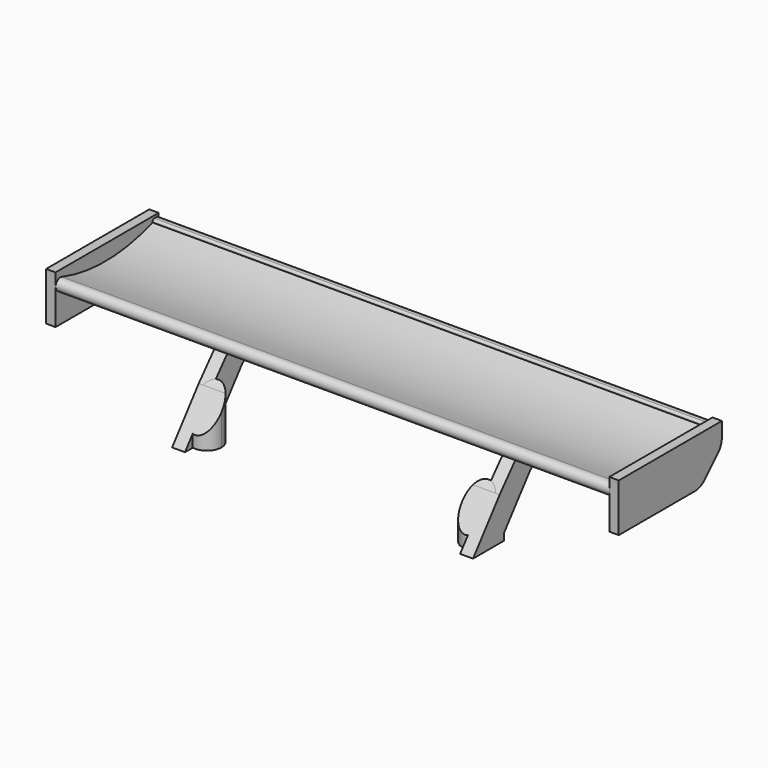
from build123d import *

# Parameters (mm, degrees)
F4_W      = 15
F4_H      = 5.6
F5_DEPTH  = 1.1
F6_SIZE   = 3.1
F7_W      = 15
F7_H      = 5.6
F8_DEPTH  = 1.1
F9_SIZE   = 3.1
F11_DEPTH = 32.2
F12_R     = 0.25
F13_R     = 2
F15_DEPTH = 1.5
F17_DEPTH = 1.5
F18_R     = 1.7
F19_DEPTH = 6.8
F22_W     = 36
F22_H     = 4
F24_R     = 0.75
F25_DEPTH = 2.5


with BuildPart() as f5:
    # F4 (on offset) → F5 (new body)
    with BuildSketch(Plane.YZ.offset(33.3)):
        with Locations((7.5, 2.8)):
            Rectangle(F4_W, F4_H)
    extrude(amount=-F5_DEPTH)

    # F6
    f6_edges = [f5.edges().sort_by_distance(p)[0] for p in [
        (32.75, 15, 0),
    ]]
    chamfer(f6_edges, length=F6_SIZE)



with BuildPart() as f8:
    # F7 (on offset) → F8 (new body)
    with BuildSketch(Plane.YZ.offset(-33.3)):
        with Locations((7.5, 2.8)):
            Rectangle(F7_W, F7_H)
    extrude(amount=F8_DEPTH)

    # F9
    f9_edges = [f8.edges().sort_by_distance(p)[0] for p in [
        (-32.75, 15, 0),
    ]]
    chamfer(f9_edges, length=F9_SIZE)


with BuildPart() as f5_1:
    add(f5.part)

    add(f8.part)  # F11 merges F8
    # F10 (on Right) → F11 (join, symmetric)
    with BuildSketch(Plane.YZ):
        with BuildLine():
            ThreePointArc((14.1, 4.9799904701), (7.5241974898, 3.7896224533), (0.9153141097, 4.7799835677))
            ThreePointArc((0.9153141097, 4.7799835677), (0.075756099, 4.4131641565), (0.3380033304, 3.5353028215))
            ThreePointArc((0.3380033304, 3.5353028215), (0.8766544844, 3.272139492), (1.4572901418, 3.1229341403))
            ThreePointArc((1.4572901418, 3.1229341403), (7.8107981998, 2.7603942388), (14.0573066811, 3.9767953297))
            ThreePointArc((14.0573066811, 3.9767953297), (14.7402257131, 4.4876667413), (15, 5.3))
            Line((15, 5.3), (14.1, 5.3))
            Line((14.1, 5.3), (14.1, 4.9799904701))
        make_face()
    extrude(amount=F11_DEPTH, both=True)

    # F12
    f12_edges = [f5_1.edges().sort_by_distance(p)[0] for p in [
        (0, 14.1, 5.3),
        (0, 15, 5.3),
    ]]
    fillet(f12_edges, radius=F12_R)

    # F13
    f13_edges = [f5_1.edges().sort_by_distance(p)[0] for p in [
        (32.75, 11.9, 0),
        (32.75, 15, 3.1),
        (-32.75, 15, 3.1),
        (-32.75, 11.9, 0),
    ]]
    fillet(f13_edges, radius=F13_R)

    # F14 (on offset) → F15 (join)
    with BuildSketch(Plane.YZ.offset(-16)):
        with BuildLine():
            ThreePointArc((10, 3.0037642772), (7.4076873546, 2.736270416), (4.8016114163, 2.7338166819))
            Line((4.8016114163, 2.7338166819), (4.8016114163, 0.7338166819))
            Line((4.8016114163, 0.7338166819), (2.4397989119, -1.9831378069))
            Line((2.4397989119, -1.9831378069), (-1.4298789153, -6.9614928532))
            Line((-1.4298789153, -6.9614928532), (3.0701210847, -6.9614928532))
            Line((3.0701210847, -6.9614928532), (3.0701210847, -6.1614928532))
            Line((3.0701210847, -6.1614928532), (6.8872222317, -1.2758261809))
            Line((6.8872222317, -1.2758261809), (10, 0.9037642772))
            Line((10, 0.9037642772), (10, 3.0037642772))
        make_face()
    extrude(amount=-F15_DEPTH)

    # F16 (on offset) → F17 (join)
    with BuildSketch(Plane.YZ.offset(16)):
        with BuildLine():
            Line((2.4397989119, -1.9831378069), (-1.4298789153, -6.9614928532))
            Line((-1.4298789153, -6.9614928532), (3.0701210847, -6.9614928532))
            Line((3.0701210847, -6.9614928532), (3.0701210847, -6.1614928532))
            Line((3.0701210847, -6.1614928532), (6.8872222317, -1.2758261809))
            Line((6.8872222317, -1.2758261809), (10, 0.9037642772))
            Line((10, 0.9037642772), (10, 3.0037642772))
            ThreePointArc((10, 3.0037642772), (7.4076873546, 2.736270416), (4.8016114163, 2.7338166819))
            Line((4.8016114163, 2.7338166819), (4.8016114163, 0.7338166819))
            Line((4.8016114163, 0.7338166819), (2.4397989119, -1.9831378069))
        make_face()
    extrude(amount=F17_DEPTH)

    # F18 (on face) → F19 (join)
    with BuildSketch(Plane(origin=(0, 0, -6.9614928532), x_dir=(1, 0, 0), z_dir=(0, 0, -1))):
        with BuildLine():
            Line((-16, -3.0434411378), (-16, 0.3031989684))
            ThreePointArc((-16, 0.3031989684), (-17.4, -1.3701210847), (-16, -3.0434411378))
        make_face()
        with BuildLine():
            ThreePointArc((-16, -3.0434411378), (-14.6091287885, -2.6739615657), (-14, -1.3701210847))
            ThreePointArc((-14, -1.3701210847), (-14.6091287885, -0.0662806036), (-16, 0.3031989684))
            Line((-16, 0.3031989684), (-16, -3.0434411378))
        make_face()
        with Locations((15.7, -1.3701210847)):
            Circle(F18_R)
    extrude(amount=-F19_DEPTH)

    # F23: sweep along a path in F20
    with BuildLine(Plane(origin=(-17.5, 0, 0), x_dir=(0, -1, 0), z_dir=(-1, 0, 0))) as f23_path:
        Line((-3.7519169699, -0.4737186464), (-2.4397989119, -1.9831378069))
        Line((-2.4397989119, -1.9831378069), (1.4298789153, -6.9614928532))
    # F22 (on face) → F23 (sweep, cut)
    with BuildSketch(Plane(origin=(0, -3.9117899018, -5.0321591222), x_dir=(1, 0, 0), z_dir=(0, 0.6137341658, 0.7895127445))):
        with Locations((0, 1.1435983825)):
            Rectangle(F22_W, F22_H)
    sweep(path=f23_path.line, transition=Transition.RIGHT, mode=Mode.SUBTRACT)

    # F24 (on face) → F25 (cut)
    with BuildSketch(Plane(origin=(0, 0, -6.9614928532), x_dir=(1, 0, 0), z_dir=(0, 0, -1))):
        with Locations((-15.7, -1.3701210847)):
            Circle(F24_R)
        with Locations((15.7, -1.3701210847)):
            Circle(F24_R)
    extrude(amount=-F25_DEPTH, mode=Mode.SUBTRACT)


solid = f5_1.part
